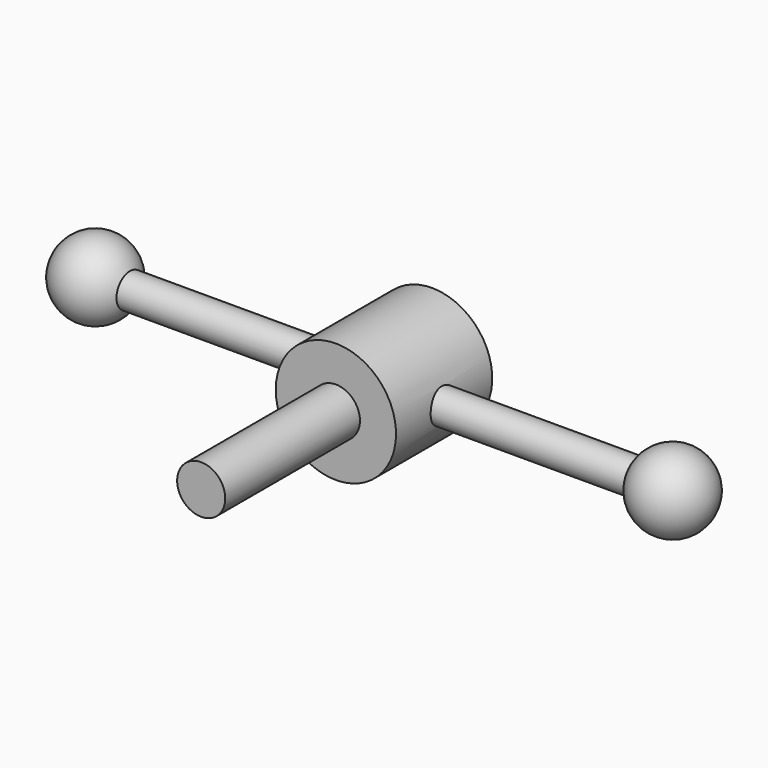
from build123d import *

# Parameters (mm, degrees)
F1_DEPTH = 15.875
F3_R     = 4.445
F4_DEPTH = 152.4
F5_R     = 6.35
F6_DEPTH = 44.45


# Not quite as in the source:
# - a pattern or mirror of a feature is missing from the dataset's text; its kind, count and spacing are read off the source's solid


with BuildPart() as f1:
    # F0 (on Front) → F1 (new body, symmetric)
    with BuildSketch(Plane.XZ):
        with BuildLine():
            ThreePointArc((92.075, 0), (76.2, 15.875), (60.325, 0))
            Line((60.325, 0), (92.075, 0))
        make_face()
        with BuildLine():
            Line((92.075, 0), (60.325, 0))
            ThreePointArc((60.325, 0), (76.2, -15.875), (92.075, 0))
        make_face()
    extrude(amount=F1_DEPTH, both=True)



with BuildPart() as f2:
    # F0 (on Front) → F2 (revolve)
    with BuildSketch(Plane.XZ):
        with BuildLine():
            ThreePointArc((-10.16, 0), (0, -10.16), (10.16, 0))
            Line((10.16, 0), (0, 0))
            Line((0, 0), (-10.16, 0))
        make_face()
    revolve(axis=Axis((76.2, 0, 0), (1, 0, 0)))


with BuildPart() as f2_copies_1:
    # F2_copies: instance of F2
    add(f2.part.mirror(Plane(origin=(76.2, 0, 0), x_dir=(0, 0, 1), z_dir=(1, 0, 0))))


with BuildPart() as f1_1:
    add(f1.part)

    add(f2.part)  # F4 merges F2

    add(f2_copies_1.part)  # F4 merges F2_copies_1
    # F3 (on Right) → F4 (join)
    with BuildSketch(Plane.YZ):
        Circle(F3_R)
    extrude(amount=F4_DEPTH)

    # F5 (on face) → F6 (join)
    with BuildSketch(Plane.XZ.offset(15.875)):
        with Locations((76.2, 0)):
            Circle(F5_R)
    extrude(amount=F6_DEPTH)


solid = f1_1.part
